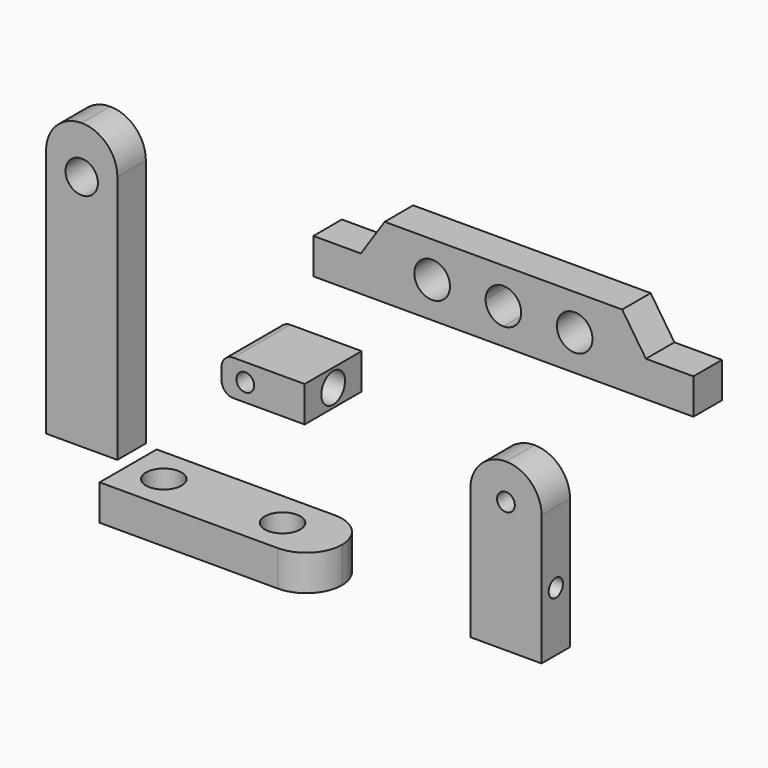
from build123d import *

# Parameters (mm, degrees)
F0_W      = 44.45
F0_H      = 19.05
F1_DEPTH  = 38.1
F3_DEPTH  = 43.18
F4_R      = 7.9375
F5_DEPTH  = 12.7
F6_R      = 6.35
F7_W      = 38.1
F7_H      = 88.9
F7_R      = 4.7625
F8_DEPTH  = 19.05
F9_R      = 4.7625
F10_DEPTH = 19.05
F11_R     = 19.04999
F12_W     = 114.3
F12_H     = 19.05
F13_DEPTH = 38.1
F14_R     = 9.525
F15_DEPTH = 101.6
F16_R     = 19.04999
F17_R     = 8.6622092444
F18_DEPTH = 19.05
F20_DEPTH = 19.05


# Not quite as in the source:
# - a fillet or chamfer is up to 0.001 mm smaller than in the source, because OpenCascade refuses the exact size


with BuildPart() as f1:
    # F0 (on Front) → F1 (new body)
    with BuildSketch(Plane.XZ):
        with Locations((-26.9059087763, 31.7358085886)):
            Rectangle(F0_W, F0_H)
    extrude(amount=-F1_DEPTH)

    # F2 (on face) → F3 (cut)
    with BuildSketch(Plane.XZ):
        with BuildLine():
            ThreePointArc((-31.6684087763, 31.7358085886), (-36.4309087763, 36.4983085886), (-41.1934087763, 31.7358085886))
            Line((-41.1934087763, 31.7358085886), (-31.6684087763, 31.7358085886))
        make_face()
        with BuildLine():
            Line((-31.6684087763, 31.7358085886), (-41.1934087763, 31.7358085886))
            ThreePointArc((-41.1934087763, 31.7358085886), (-36.4309087763, 26.9733085886), (-31.6684087763, 31.7358085886))
        make_face()
    extrude(amount=-F3_DEPTH, mode=Mode.SUBTRACT)

    # F4 (on face) → F5 (cut)
    with BuildSketch(Plane.YZ.offset(-4.6809087763)):
        with Locations((19.05, 31.7358085886)):
            Circle(F4_R)
    extrude(amount=-F5_DEPTH, mode=Mode.SUBTRACT)

    # F6
    f6_edges = [f1.edges().sort_by_distance(p)[0] for p in [
        (-49.130909, 19.05, 41.260809),
        (-49.130909, 19.05, 22.210809),
    ]]
    fillet(f6_edges, radius=F6_R)


with BuildPart() as f8:
    # F7 (on Front) → F8 (new body)
    with BuildSketch(Plane.XZ):
        with Locations((118.1868945239, 8.0456975847)):
            Rectangle(F7_W, F7_H)
        with Locations((118.1868945239, 33.4456975847)):
            Circle(F7_R, mode=Mode.SUBTRACT)
    extrude(amount=F8_DEPTH)

    # F9 (on face) → F10 (cut)
    with BuildSketch(Plane.YZ.offset(137.2368945239)):
        with Locations((-9.525, -4.6543024153)):
            Circle(F9_R)
    extrude(amount=-F10_DEPTH, mode=Mode.SUBTRACT)

    # F11 (radius 19.05 in the source; OpenCascade refuses exactly that, so slightly less here)
    f11_edges = [f8.edges().sort_by_distance(p)[0] for p in [
        (137.236895, -9.525, 52.495698),
        (99.136895, -9.525, 52.495698),
    ]]
    fillet(f11_edges, radius=F11_R)


with BuildPart() as f13:
    # F12 (on Front) → F13 (new body)
    with BuildSketch(Plane.XZ):
        with Locations((-57.15, -50.1792910555)):
            Rectangle(F12_W, F12_H)
    extrude(amount=-F13_DEPTH)

    # F14 (on face) → F15 (cut)
    with BuildSketch(Plane.XY.offset(-40.6542910555)):
        with Locations((-95.25, 19.05)):
            Circle(F14_R)
        with Locations((-31.75, 19.05)):
            Circle(F14_R)
    extrude(amount=-F15_DEPTH, mode=Mode.SUBTRACT)

    # F16 (radius 19.05 in the source; OpenCascade refuses exactly that, so slightly less here)
    f16_edges = [f13.edges().sort_by_distance(p)[0] for p in [
        (0, 38.1, -50.179291),
        (0, 0, -50.179291),
    ]]
    fillet(f16_edges, radius=F16_R)


with BuildPart() as f18:
    # F17 (on Front) → F18 (new body)
    with BuildSketch(Plane.XZ):
        with BuildLine():
            Line((-127.7065266967, 119.0175100861), (-127.7065266967, -14.3324899139))
            Line((-127.7065266967, -14.3324899139), (-89.6065266967, -14.3324899139))
            Line((-89.6065266967, -14.3324899139), (-89.6065266967, 119.0175100861))
            ThreePointArc((-89.6065266967, 119.0175100861), (-95.1861425151, 132.4878942677), (-108.6565266967, 138.0675100861))
            ThreePointArc((-108.6565266967, 138.0675100861), (-122.1269108783, 132.4878942677), (-127.7065266967, 119.0175100861))
        make_face()
        with Locations((-108.6565266967, 112.6675100861)):
            Circle(F17_R, mode=Mode.SUBTRACT)
    extrude(amount=F18_DEPTH)


with BuildPart() as f20:
    # F19 (on Front) → F20 (new body)
    with BuildSketch(Plane.XZ):
        with BuildLine():
            Line((101.6, 131.5424591149), (38.1, 131.5424591149))
            Line((38.1, 131.5424591149), (25.4, 112.4924591149))
            Line((25.4, 112.4924591149), (53.975, 112.4924591149))
            ThreePointArc((53.975, 112.4924591149), (63.5, 122.0174591149), (73.025, 112.4924591149))
            Line((73.025, 112.4924591149), (92.075, 112.4924591149))
            ThreePointArc((92.075, 112.4924591149), (94.8648079092, 119.2276512057), (101.6, 122.0174591149))
            Line((101.6, 122.0174591149), (101.6, 131.5424591149))
        make_face()
        with BuildLine():
            Line((165.1, 131.5424591149), (101.6, 131.5424591149))
            Line((101.6, 131.5424591149), (101.6, 122.0174591149))
            ThreePointArc((101.6, 122.0174591149), (108.3351920908, 119.2276512057), (111.125, 112.4924591149))
            Line((111.125, 112.4924591149), (130.175, 112.4924591149))
            ThreePointArc((130.175, 112.4924591149), (139.7, 122.0174591149), (149.225, 112.4924591149))
            Line((149.225, 112.4924591149), (177.8, 112.4924591149))
            Line((177.8, 112.4924591149), (165.1, 131.5424591149))
        make_face()
        with BuildLine():
            Line((53.975, 112.4924591149), (25.4, 112.4924591149))
            Line((25.4, 112.4924591149), (0, 112.4924591149))
            Line((0, 112.4924591149), (0, 93.4424591149))
            Line((0, 93.4424591149), (101.6, 93.4424591149))
            Line((101.6, 93.4424591149), (101.6, 102.9674591149))
            ThreePointArc((101.6, 102.9674591149), (94.8648079092, 105.7572670241), (92.075, 112.4924591149))
            Line((92.075, 112.4924591149), (73.025, 112.4924591149))
            ThreePointArc((73.025, 112.4924591149), (63.5, 102.9674591149), (53.975, 112.4924591149))
        make_face()
        with BuildLine():
            Line((203.2, 112.4924591149), (177.8, 112.4924591149))
            Line((177.8, 112.4924591149), (149.225, 112.4924591149))
            ThreePointArc((149.225, 112.4924591149), (139.7, 102.9674591149), (130.175, 112.4924591149))
            Line((130.175, 112.4924591149), (111.125, 112.4924591149))
            ThreePointArc((111.125, 112.4924591149), (108.3351920908, 105.7572670241), (101.6, 102.9674591149))
            Line((101.6, 102.9674591149), (101.6, 93.4424591149))
            Line((101.6, 93.4424591149), (203.2, 93.4424591149))
            Line((203.2, 93.4424591149), (203.2, 112.4924591149))
        make_face()
    extrude(amount=-F20_DEPTH)


solid = Compound([f1.part, f8.part, f13.part, f18.part, f20.part])
